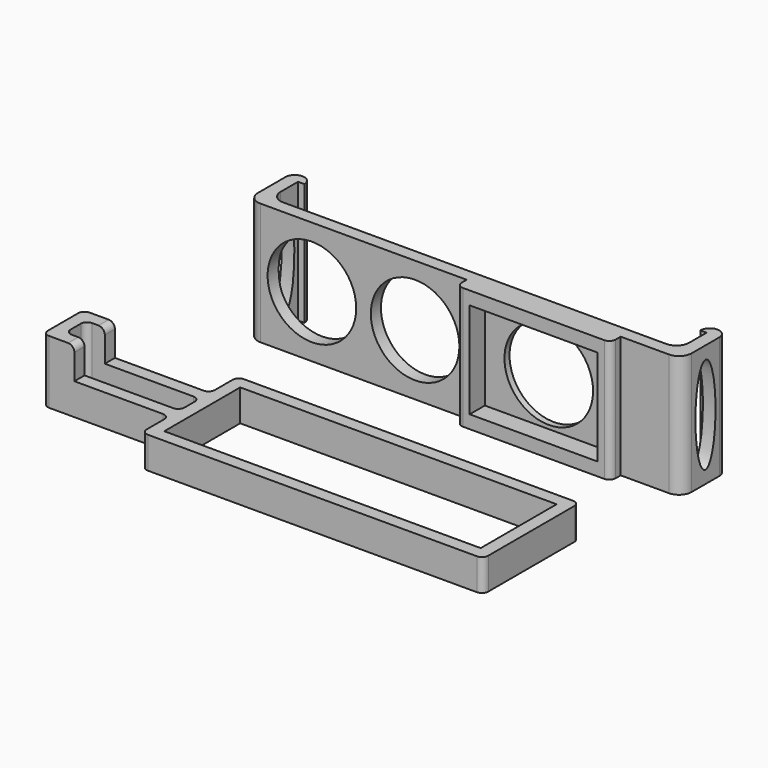
from build123d import *

# Parameters (mm, degrees)
F2_DEPTH  = 19.3
F5_DEPTH  = 68.571
F7_R      = 1
F6_W      = 18
F6_H      = 4
F6_W_2    = 50
F6_H_2    = 15
F8_DEPTH  = 5
F10_DEPTH = 5
F11_R     = 1
F3_W      = 20.2
F3_H      = 15.16
F12_DEPTH = 3
F13_R     = 7
F14_R     = 7
F15_DEPTH = 8.951


with BuildPart() as f2:
    # F1 (on Top) → F2 (new body)
    with BuildSketch(Plane.XY):
        with BuildLine():
            Line((24.67, -1), (32.285, -1))
            ThreePointArc((32.285, -1), (33.6992135624, -0.4142135624), (34.285, 1))
            Line((34.285, 1), (34.285, 6.45))
            ThreePointArc((34.285, 6.45), (32.785, 7.95), (31.285, 6.45))
            Line((31.285, 6.45), (32.285, 6.45))
            Line((32.285, 6.45), (32.285, 3))
            ThreePointArc((32.285, 3), (31.6992135624, 1.5857864376), (30.285, 1))
            Line((30.285, 1), (24.67, 1))
            Line((24.67, 1), (24.67, -1))
        make_face()
        Polygon((24.67, -3), (24.67, -1), (24.67, 1), (12.17, 1), (0.33, 1), (0.33, -1), (0.33, -3), align=None)
        with BuildLine():
            Line((0.33, -1), (0.33, 1))
            Line((0.33, 1), (-12.17, 1))
            Line((-12.17, 1), (-30.285, 1))
            ThreePointArc((-30.285, 1), (-31.6992135624, 1.5857864376), (-32.285, 3))
            Line((-32.285, 3), (-32.285, 6.45))
            Line((-32.285, 6.45), (-31.285, 6.45))
            ThreePointArc((-31.285, 6.45), (-32.785, 7.95), (-34.285, 6.45))
            Line((-34.285, 6.45), (-34.285, 1))
            ThreePointArc((-34.285, 1), (-33.6992135624, -0.4142135624), (-32.285, -1))
            Line((-32.285, -1), (-12.17, -1))
            Line((-12.17, -1), (0.33, -1))
        make_face()
    extrude(amount=F2_DEPTH)

    # F4 (on face) → F5 (cut, through all)
    with BuildSketch(Plane.YZ.offset(34.285)):
        with BuildLine():
            add(Edge.make_bspline(
                [(3.725, 17.3), (0.2608983849, 17.3), (1.9929491924, 5.825), (3.725, -5.65), (5.4570508076, 5.825), (7.1891016151, 17.3), (3.725, 17.3)],
                knots=[0, 0, 0, 2.0943951024, 2.0943951024, 4.1887902048, 4.1887902048, 6.2831853072, 6.2831853072, 6.2831853072], degree=2, weights=[1, 0.5, 1, 0.5, 1, 0.5, 1]))
        make_face()
    extrude(amount=-F5_DEPTH, mode=Mode.SUBTRACT)

    # F7
    f7_edges = [f2.edges().sort_by_distance(p)[0] for p in [
        (0.33, -3, 9.65),
        (24.67, -3, 9.65),
    ]]
    fillet(f7_edges, radius=F7_R)

    # F3 (on face) → F12 (cut)
    with BuildSketch(Plane.XZ.offset(3)):
        with Locations((12.5, 9.65)):
            Rectangle(F3_W, F3_H)
    extrude(amount=-F12_DEPTH, mode=Mode.SUBTRACT)

    # F13 (on face) + F14 (on face) → F15 (cut, through all)
    with BuildSketch(Plane.XZ.offset(1)):
        with Locations((-24.13125, 9.65)):
            Circle(F13_R)
        with Locations((-7.82375, 9.65)):
            Circle(F13_R)
    with BuildSketch(Plane.XZ):
        with Locations((12.5, 9.65)):
            Circle(F14_R)
    extrude(amount=-F15_DEPTH, mode=Mode.SUBTRACT)


with BuildPart() as f8:
    # F6 (on Top) → F8 (new body)
    with BuildSketch(Plane.XY):
        Polygon((-22.6870492548, -30.9672894628), (-22.6870492548, -36.4672894628), (31.3129507452, -36.4672894628), (31.3129507452, -17.4672894628), (-22.6870492548, -17.4672894628), (-22.6870492548, -22.9672894628), (-42.6870492548, -22.9672894628), (-42.6870492548, -30.9672894628), align=None)
        with Locations((-31.6870492548, -26.9672894628)):
            Rectangle(F6_W, F6_H, mode=Mode.SUBTRACT)
        with Locations((4.3129507452, -26.9672894628)):
            Rectangle(F6_W_2, F6_H_2, mode=Mode.SUBTRACT)
    extrude(amount=F8_DEPTH)

    # F9 (on face) → F10 (join)
    with BuildSketch(Plane.XY.offset(5)):
        Polygon((-37.6870492548, -22.9672894628), (-42.6870492548, -22.9672894628), (-42.6870492548, -30.9672894628), (-37.6870492548, -30.9672894628), (-37.6870492548, -28.9672894628), (-40.6870492548, -28.9672894628), (-40.6870492548, -24.9672894628), (-37.6870492548, -24.9672894628), align=None)
    extrude(amount=F10_DEPTH)

    # F11
    f11_edges = [f8.edges().sort_by_distance(p)[0] for p in [
        (-37.687049, -29.967289, 10),
        (-37.687049, -23.967289, 10),
        (-22.687049, -36.467289, 2.5),
        (31.312951, -36.467289, 2.5),
        (31.312951, -17.467289, 2.5),
        (-42.687049, -30.967289, 5),
        (-42.687049, -22.967289, 5),
        (-22.687049, -22.967289, 2.5),
        (-22.687049, -17.467289, 2.5),
        (-22.687049, -30.967289, 2.5),
        (-40.687049, -24.967289, 5),
        (-40.687049, -28.967289, 5),
        (-22.687049, -24.967289, 2.5),
        (-22.687049, -28.967289, 2.5),
    ]]
    fillet(f11_edges, radius=F11_R)


solid = Compound([f2.part, f8.part])
